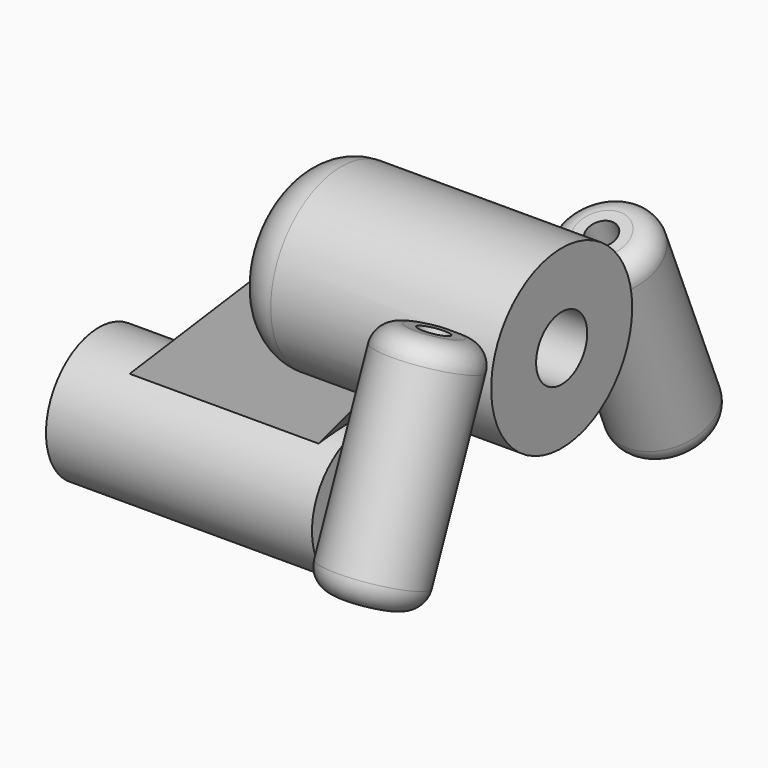
from build123d import *

# Parameters (mm, degrees)
F0_R      = 4
F1_DEPTH  = 2
F2_R      = 4
F2_R_2    = 1.45
F3_DEPTH  = 10
F5_DEPTH  = 1.5
F8_R      = 3
F9_DEPTH  = 12.07
F10_R     = 0.75
F11_DEPTH = 25
F13_R     = 2
F14_R     = 2.15
F14_R_2   = 0.65
F15_DEPTH = 10
F16_R     = 0.99999


# Not quite as in the source:
# - a fillet or chamfer is up to 0.001 mm smaller than in the source, because OpenCascade refuses the exact size


with BuildPart() as f1:
    # F0 (on Right) → F1 (new body)
    with BuildSketch(Plane.YZ):
        Circle(F0_R)
    extrude(amount=F1_DEPTH)

    # F2 (on face) → F3 (join)
    with BuildSketch(Plane.YZ.offset(2)):
        Circle(F2_R)
        Circle(F2_R_2, mode=Mode.SUBTRACT)
    extrude(amount=F3_DEPTH)

    # F4 (on Front) → F5 (join, symmetric)
    with BuildSketch(Plane.XZ):
        Polygon((0, -3), (0, 0), (-9, -9), (0, -9), (5, -3), align=None)
    extrude(amount=F5_DEPTH, both=True)

    # F8 (on plane+point) → F9 (join)
    with BuildSketch(Plane.YZ.offset(-9)):
        with Locations((0, -9)):
            Circle(F8_R)
    extrude(amount=F9_DEPTH)

    # F10 (on face) → F11 (cut)
    with BuildSketch(Plane(origin=(-9, 0, 0), x_dir=(0, -1, 0), z_dir=(-1, 0, 0))):
        with Locations((0, -9)):
            Circle(F10_R)
    extrude(amount=-F11_DEPTH, mode=Mode.SUBTRACT)

    # F13
    f13_edges = [f1.edges().sort_by_distance(p)[0] for p in [
        (0, -2.236068, 3.316625),
    ]]
    fillet(f13_edges, radius=F13_R)

    # F14 (on face) → F15 (join)
    with BuildSketch(Plane(origin=(0, 0, 0), x_dir=(1, 0, 0), z_dir=(0, -0.3826834324, -0.9238795325))):
        with Locations((10, 5.15)):
            Circle(F14_R)
        with Locations((10, 5.15)):
            Circle(F14_R_2, mode=Mode.SUBTRACT)
    extrude(amount=F15_DEPTH)

    # F16 (radius 1 in the source; OpenCascade refuses exactly that, so slightly less here)
    f16_edges = [f1.edges().sort_by_distance(p)[0] for p in [
        (7.85, -8.584814, -7.267976),
        (9.401322, -6.665759, 2.761048),
    ]]
    fillet(f16_edges, radius=F16_R)

    # F17: F1 across plane


with BuildPart() as f1_1:
    add(f1.part)
    add(f1.part.mirror(Plane.XZ))


solid = f1_1.part
